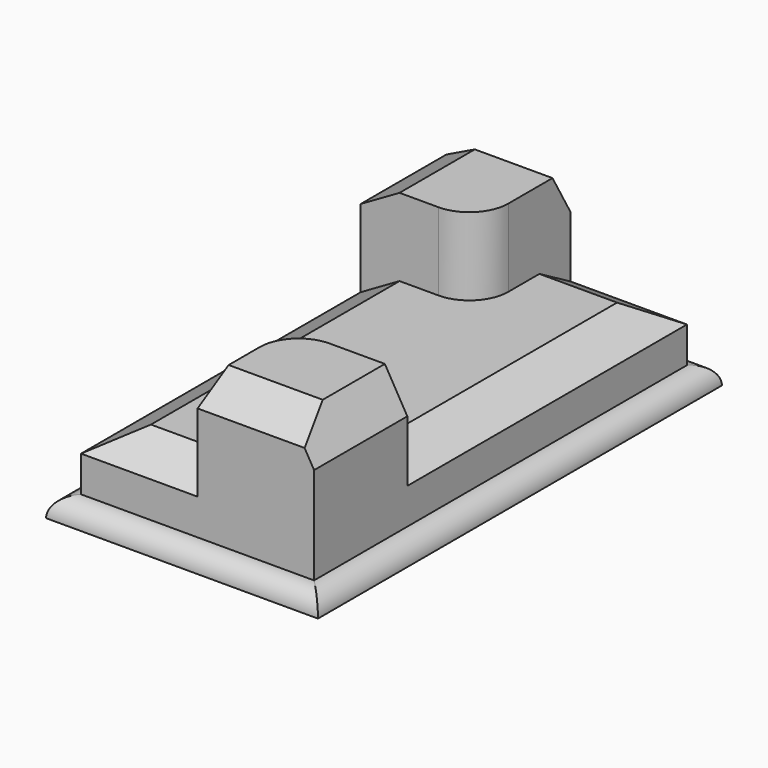
from build123d import *

# Parameters (mm, degrees)
F1_DEPTH    = 6.35
F2_DEPTH    = 25.4
F3_DEPTH    = 50.8
F4_C1_SIZE2 = 12.7
F4_C1_SIZE  = 7.3323484187
F4_C2_SIZE2 = 12.7
F4_C2_SIZE  = 7.3323484187
F4_C3_SIZE2 = 7.3323484187
F4_C3_SIZE  = 12.7
F4_C4_SIZE2 = 12.7
F4_C4_SIZE  = 7.3323484187
F4_C5_SIZE2 = 12.7
F4_C5_SIZE  = 7.3323484187
F4_C6_SIZE2 = 12.7
F4_C6_SIZE  = 7.3323484187
F4_C7_SIZE2 = 12.7
F4_C7_SIZE  = 7.3323484187
F4_C8_SIZE2 = 12.7
F4_C8_SIZE  = 7.3323484187
F5_R        = 6.34999


# Not quite as in the source:
# - a fillet or chamfer is up to 0.001 mm smaller than in the source, because OpenCascade refuses the exact size


with BuildPart() as f1:
    # F0 (on Top) → F1 (new body)
    with BuildSketch(Plane.XY):
        Polygon((-38.1, 38.1), (-38.1, 76.2), (0, 76.2), (38.1, 76.2), (38.1, 82.55), (-44.45, 82.55), (-44.45, -82.55), (-38.1, -82.55), (-38.1, -76.2), align=None)
        Polygon((38.1, 82.55), (38.1, 76.2), (38.1, -38.1), (38.1, -76.2), (0, -76.2), (-38.1, -76.2), (-38.1, -82.55), (44.45, -82.55), (44.45, 82.55), align=None)
    extrude(amount=F1_DEPTH)

    # F0 (on Top) → F2 (join)
    with BuildSketch(Plane.XY):
        with BuildLine():
            Line((38.1, 76.2), (0, 76.2))
            Line((0, 76.2), (0, 50.8))
            ThreePointArc((0, 50.8), (-3.7197438789, 41.8197438789), (-12.7, 38.1))
            Line((-12.7, 38.1), (-38.1, 38.1))
            Line((-38.1, 38.1), (-38.1, -76.2))
            Line((-38.1, -76.2), (0, -76.2))
            Line((0, -76.2), (0, -50.8))
            ThreePointArc((0, -50.8), (3.7197438789, -41.8197438789), (12.7, -38.1))
            Line((12.7, -38.1), (38.1, -38.1))
            Line((38.1, -38.1), (38.1, 76.2))
        make_face()
    extrude(amount=F2_DEPTH)

    # F0 (on Top) → F3 (join)
    with BuildSketch(Plane.XY):
        with BuildLine():
            Line((0, 76.2), (-38.1, 76.2))
            Line((-38.1, 76.2), (-38.1, 38.1))
            Line((-38.1, 38.1), (-12.7, 38.1))
            ThreePointArc((-12.7, 38.1), (-3.7197438789, 41.8197438789), (0, 50.8))
            Line((0, 50.8), (0, 76.2))
        make_face()
        with BuildLine():
            Line((38.1, -76.2), (38.1, -38.1))
            Line((38.1, -38.1), (12.7, -38.1))
            ThreePointArc((12.7, -38.1), (3.7197438789, -41.8197438789), (0, -50.8))
            Line((0, -50.8), (0, -76.2))
            Line((0, -76.2), (38.1, -76.2))
        make_face()
    extrude(amount=F3_DEPTH)

    # F4: chamfer of 12.7 x 7.3323484187 on 8 edges, made by hand

    # F4_c1
    f4_c1_edges = [f1.edges().sort_by_distance(p)[0] for p in [
        (-19.05, -76.2, 25.4),
    ]]
    f4_c1_side = f1.faces().sort_by_distance((-19.05, -76.2, 25.2533530316))[0]
    chamfer(f4_c1_edges, length=F4_C1_SIZE, length2=F4_C1_SIZE2, reference=f4_c1_side)

    # F4_c2
    f4_c2_edges = [f1.edges().sort_by_distance(p)[0] for p in [
        (19.05, -76.2, 50.8),
    ]]
    f4_c2_side = f1.faces().sort_by_distance((19.05, -76.2, 50.6533530316))[0]
    chamfer(f4_c2_edges, length=F4_C2_SIZE, length2=F4_C2_SIZE2, reference=f4_c2_side)

    # F4_c3
    f4_c3_edges = [f1.edges().sort_by_distance(p)[0] for p in [
        (38.1, -50.8, 50.8),
    ]]
    f4_c3_side = f1.faces().sort_by_distance((38.1, -50.8, 50.6533530316))[0]
    chamfer(f4_c3_edges, length=F4_C3_SIZE, length2=F4_C3_SIZE2, reference=f4_c3_side)

    # F4_c4
    f4_c4_edges = [f1.edges().sort_by_distance(p)[0] for p in [
        (38.1, 19.05, 25.4),
    ]]
    f4_c4_side = f1.faces().sort_by_distance((38.1, 19.05, 25.2533530316))[0]
    chamfer(f4_c4_edges, length=F4_C4_SIZE, length2=F4_C4_SIZE2, reference=f4_c4_side)

    # F4_c5
    f4_c5_edges = [f1.edges().sort_by_distance(p)[0] for p in [
        (12.7, 76.2, 25.4),
    ]]
    f4_c5_side = f1.faces().sort_by_distance((12.7, 76.2, 25.2533530316))[0]
    chamfer(f4_c5_edges, length=F4_C5_SIZE, length2=F4_C5_SIZE2, reference=f4_c5_side)

    # F4_c6
    f4_c6_edges = [f1.edges().sort_by_distance(p)[0] for p in [
        (-38.1, -12.7, 25.4),
    ]]
    f4_c6_side = f1.faces().sort_by_distance((-38.1, -12.7, 25.2533530316))[0]
    chamfer(f4_c6_edges, length=F4_C6_SIZE, length2=F4_C6_SIZE2, reference=f4_c6_side)

    # F4_c7
    f4_c7_edges = [f1.edges().sort_by_distance(p)[0] for p in [
        (-19.05, 76.2, 50.8),
    ]]
    f4_c7_side = f1.faces().sort_by_distance((-19.05, 76.0533530316, 50.8))[0]
    chamfer(f4_c7_edges, length=F4_C7_SIZE, length2=F4_C7_SIZE2, reference=f4_c7_side)

    # F4_c8
    f4_c8_edges = [f1.edges().sort_by_distance(p)[0] for p in [
        (-38.1, 53.4838257906, 50.8),
    ]]
    f4_c8_side = f1.faces().sort_by_distance((-38.1, 53.4838257906, 50.6533530316))[0]
    chamfer(f4_c8_edges, length=F4_C8_SIZE, length2=F4_C8_SIZE2, reference=f4_c8_side)

    # F5 (radius 6.35 in the source; OpenCascade refuses exactly that, so slightly less here)
    f5_edges = [f1.edges().sort_by_distance(p)[0] for p in [
        (-44.45, 0, 6.35),
        (0, 82.55, 6.35),
        (44.45, 0, 6.35),
        (0, -82.55, 6.35),
    ]]
    fillet(f5_edges, radius=F5_R)


solid = f1.part
